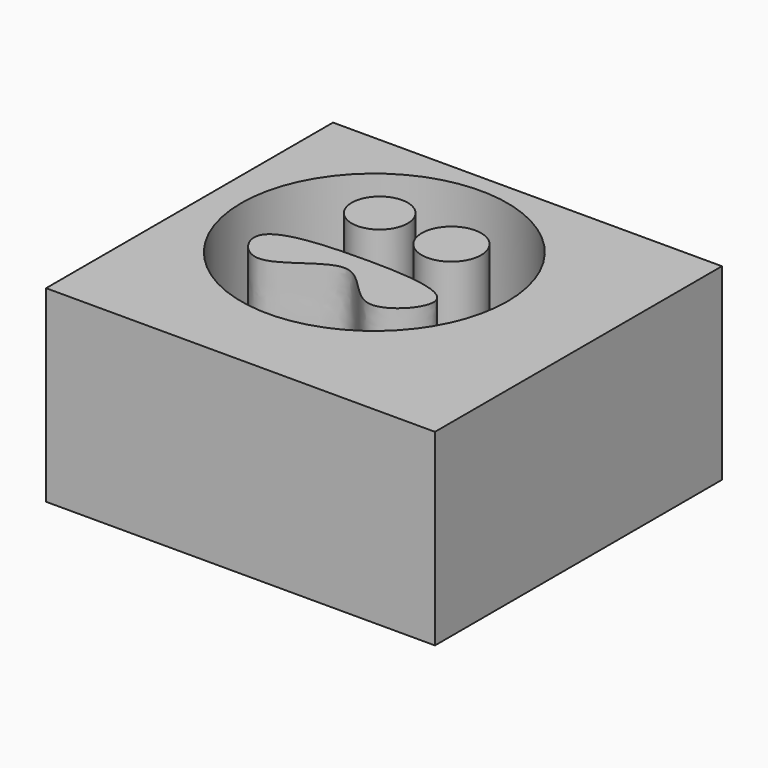
from build123d import *

# Parameters (mm, degrees)
F0_W     = 52.5235719979
F0_H     = 48.4414305538
F1_DEPTH = 25.4
F3_R     = 17.9806924125
F3_R_2   = 3.780727698
F3_R_3   = 4.0181404967
F6_DEPTH = 27.432
F7_DEPTH = 18.288


# Not quite as in the source:
# - the program builds the solid bodies; features that only make, move or delete a surface that nothing else refers to are left out


with BuildPart() as f1:
    # F0 (on Top) → F1 (new body)
    with BuildSketch(Plane.XY):
        with Locations((4.3542869389, 0.9524999186)):
            Rectangle(F0_W, F0_H)
    extrude(amount=F1_DEPTH)

    # F3 (on face) → F6 (cut)
    with BuildSketch(Plane.XY.offset(25.4)):
        with Locations((0, 4.7625000589)):
            Circle(F3_R)
        with Locations((-5.1515786909, 12.1103571728)):
            Circle(F3_R_2, mode=Mode.SUBTRACT)
        with Locations((5.1898504607, 11.2939290702)):
            Circle(F3_R_3, mode=Mode.SUBTRACT)
    extrude(amount=-F6_DEPTH, mode=Mode.SUBTRACT)


with BuildPart() as f7:
    # F4 (on face) → F7 (new body)
    with BuildSketch(Plane.XY.offset(25.4)):
        with BuildLine():
            add(Edge.make_bspline(
                [(-11.9551504031, 0), (-11.3374873906, 2.3918507841), (-0.1404740389, 3.2569434634), (16.0461571526, 2.2516272688), (6.2552175699, -8.3932651273), (0.4505515588, 4.2969461524), (-8.3923398431, -7.1268055014), (-12.3538703235, -1.5440111115), (-11.9551504031, 0)],
                knots=[0, 0, 0, 0, 0.1957909913, 0.3918782168, 0.5378469307, 0.701092352, 0.873611068, 1, 1, 1, 1], degree=3))
        make_face()
    extrude(amount=-F7_DEPTH)


solid = Compound([f1.part, f7.part])
